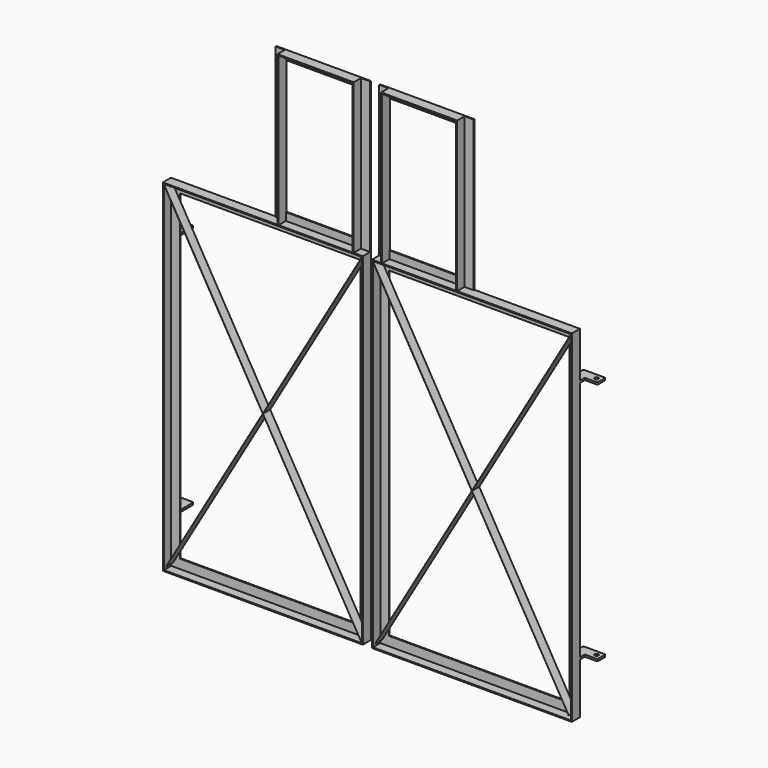
from build123d import *

# Parameters (mm, degrees)
F0_W      = 985
F0_H      = 1685
F1_DEPTH  = 50
F2_T      = -5
F3_W      = 890
F3_H      = 1585
F4_DEPTH  = 50.001
F5_W      = 375
F5_H      = 740
F6_DEPTH  = 50
F7_T      = -5
F8_W      = 365
F8_H      = 660
F9_DEPTH  = 5.001
F10_W     = 45
F10_H     = 5
F11_DEPTH = 740
F13_DEPTH = 45
F16_W     = 47.5
F16_H     = 10
F17_DEPTH = 80
F18_W     = 50
F18_H     = 10
F19_DEPTH = 62.5
F20_R     = 9
F21_DEPTH = 1460.001
F22_R     = 5


# Not quite as in the source:
# - a shell that OpenCascade refuses in one call is made with other operations: the cavity is built on its own and cut out


with BuildPart() as f1:
    # F0 (on Front) → F1 (new body)
    with BuildSketch(Plane.XZ):
        Rectangle(F0_W, F0_H)
    extrude(amount=F1_DEPTH)

    # F2
    f2_openings = [f1.faces().sort_by_distance(p)[0] for p in [
        (0, -50, 0),
    ]]
    offset(amount=F2_T, openings=f2_openings)

    # F3 (on face) → F4 (cut, through all)
    with BuildSketch(Plane.XZ.offset(50)):
        Rectangle(F3_W, F3_H)
    extrude(amount=-F4_DEPTH, mode=Mode.SUBTRACT)

    # F5 (on Front) → F6 (join)
    with BuildSketch(Plane.XZ):
        with Locations((260, 1212.5)):
            Rectangle(F5_W, F5_H)
    extrude(amount=F6_DEPTH)

    # F7: a shell. OpenCascade refuses it in one call, so the cavity is built on its own and cut out:
    # the body offset inwards by the wall thickness, plus a prism from it out through each open face.
    f7_core = offset(f1.part, amount=F7_T, kind=Kind.INTERSECTION, mode=Mode.PRIVATE)
    f7_exits = [f7_core.faces().sort_by_distance(p)[0] for p in [
        (260, -45, 1210),
    ]]
    add(f7_core, mode=Mode.SUBTRACT)
    extrude(f7_exits, amount=-F7_T, mode=Mode.SUBTRACT)

    # F8 (on face) → F9 (cut, through all)
    with BuildSketch(Plane.XZ.offset(5)):
        with Locations((260, 1210)):
            Rectangle(F8_W, F8_H)
    extrude(amount=-F9_DEPTH, mode=Mode.SUBTRACT)

    # F10 (on face) → F11 (join)
    with BuildSketch(Plane.XY.offset(842.5)):
        with Locations((50, -2.5)):
            Rectangle(F10_W, F10_H)
        with Locations((470, -2.5)):
            Rectangle(F10_W, F10_H)
    extrude(amount=F11_DEPTH)

    # F16 (on face) → F17 (join)
    with BuildSketch(Plane(origin=(0, 0, 0), x_dir=(-1, 0, 0), z_dir=(0, 1, 0))):
        with Locations((468.75, -587.5)):
            Rectangle(F16_W, F16_H)
        with Locations((468.75, 612.5)):
            Rectangle(F16_W, F16_H)
    extrude(amount=F17_DEPTH)

    # F18 (on face) → F19 (join)
    with BuildSketch(Plane(origin=(-492.5, 0, 0), x_dir=(0, -1, 0), z_dir=(-1, 0, 0))):
        with Locations((-55, 612.5)):
            Rectangle(F18_W, F18_H)
        with Locations((-55, -587.5)):
            Rectangle(F18_W, F18_H)
    extrude(amount=F19_DEPTH)

    # F20 (on face) → F21 (cut, through all)
    with BuildSketch(Plane.XY.offset(617.5)):
        with Locations((-530, 55)):
            Circle(F20_R)
    extrude(amount=-F21_DEPTH, mode=Mode.SUBTRACT)

    # F22
    f22_edges = [f1.edges().sort_by_distance(p)[0] for p in [
        (-445, 80, 612.5),
        (-555, 80, 612.5),
        (-555, 30, 612.5),
        (-555, 30, -587.5),
        (-555, 80, -587.5),
        (-445, 80, -587.5),
    ]]
    fillet(f22_edges, radius=F22_R)


with BuildPart() as f13:
    # F12 (on face) → F13 (new body)
    with BuildSketch(Plane.XZ.offset(5)):
        Polygon((487.8614675759, -837.5), (487.5, -836.87971525), (487.5, -837.5), align=None)
    extrude(amount=F13_DEPTH)


with BuildPart() as f13b:
    # F12 (on face) → F13, piece 2 (new body)
    with BuildSketch(Plane.XZ.offset(5)):
        Polygon((487.5, -836.8550058622), (477.1365219459, -819.0958037114), (487.5, -836.87971525), align=None)
    extrude(amount=F13_DEPTH)


with BuildPart() as f13c:
    # F12 (on face) → F13, piece 3 (new body)
    with BuildSketch(Plane.XZ.offset(5)):
        Polygon((477.1365219459, -819.0958037114), (-487.5, 836.2375200634), (-487.5, 837.5), (-489.5788806122, 837.5), align=None)
    extrude(amount=F13_DEPTH)


with BuildPart() as f14_1:
    # F14: instance of F13c
    add(f13c.part.mirror(Plane.YZ))


with BuildPart() as f23_1:
    # F23: instance of F1
    add(f1.part.mirror(Plane.YZ.offset(515)))


with BuildPart() as f23_2:
    # F23: instance of F13c
    add(f13c.part.mirror(Plane.YZ.offset(515)))


with BuildPart() as f23_3:
    # F23: instance of F14_1
    add(f14_1.part.mirror(Plane.YZ.offset(515)))


solid = Compound([f1.part, f13.part, f13b.part, f13c.part, f14_1.part, f23_1.part, f23_2.part, f23_3.part])
